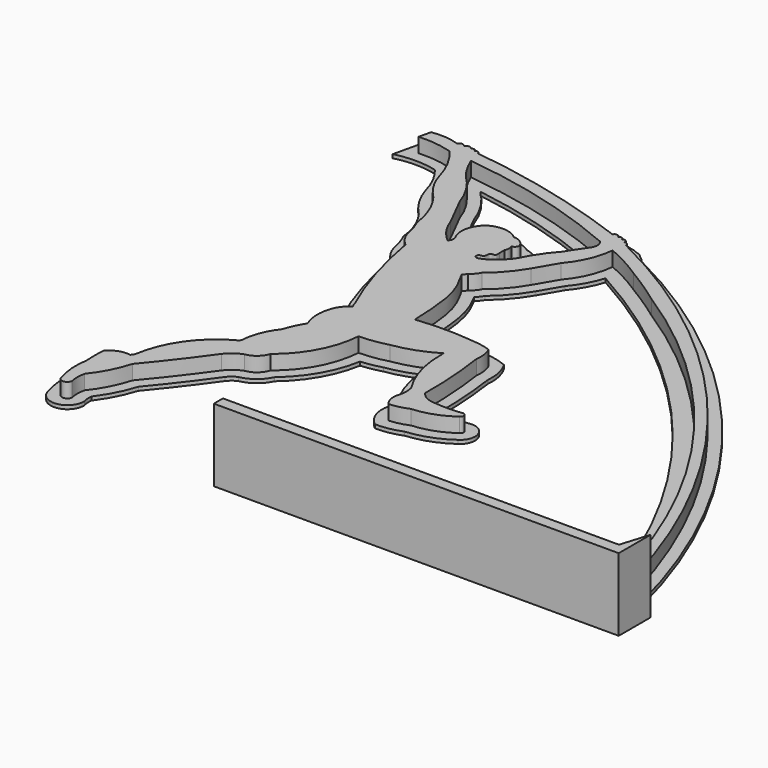
from build123d import *

# Parameters (mm, degrees)
F1_DEPTH = 2.5
F2_DEPTH = 0.5
F3_DEPTH = 10


# Not quite as in the source:
# - ends of sketch curves that miss each other by under 0.0002 mm in the source are joined
# - the dataset's text gives a spline's control points without its knots; the knots are read off the source's solid


with BuildPart() as f1:
    # F0 (on Top) → F1 (new body)
    with BuildSketch(Plane.XY):
        with BuildLine():
            ThreePointArc((-39.8229367736, 44.1013294606), (-37.4652443011, 44.0384179647), (-35.1560073833, 43.5587342062))
            ThreePointArc((-35.1560073833, 43.5587342062), (-33.4579822766, 41.1148254491), (-32.3751845495, 38.3429076368))
            ThreePointArc((-32.3751845495, 38.3429076368), (-31.3502645154, 36.0621986154), (-29.7918598256, 34.1068292029))
            ThreePointArc((-29.7918598256, 34.1068292029), (-28.2885518159, 31.4484118208), (-27.5291783241, 28.4902925114))
            ThreePointArc((-27.5291783241, 28.4902925114), (-26.9990197914, 27.1071797984), (-26.6612432485, 25.6649676596))
            ThreePointArc((-26.6612432485, 25.6649676596), (-26.0965046118, 24.5488660128), (-25.2444654097, 23.633092126))
            ThreePointArc((-25.2444654097, 23.633092126), (-23.5305341122, 16.3912786142), (-20.9041361566, 9.4282722799))
            ThreePointArc((-20.9041361566, 9.4282722799), (-20.8326707518, 9.1409651891), (-20.6576495277, 8.902176078))
            ThreePointArc((-20.6576495277, 8.902176078), (-21.6263146631, 8.0093254226), (-22.2124983376, 6.8295444526))
            ThreePointArc((-22.2124983376, 6.8295444526), (-22.4900033885, 4.788054511), (-22.0261043394, 2.7806960709))
            ThreePointArc((-22.0261043394, 2.7806960709), (-22.7702995051, 1.4335862053), (-23.3300869888, 0))
            ThreePointArc((-23.3300869888, 0), (-24.5116215298, -2.0072475649), (-25.10167519, -4.260446033))
            ThreePointArc((-25.10167519, -4.260446033), (-25.2008110189, -4.7928851197), (-25.6555593813, -5.0870334166))
            ThreePointArc((-25.6555593813, -5.0870334166), (-29.86125263, -8.9331377893), (-31.9792483024, -14.224117744))
            ThreePointArc((-31.9792483024, -14.224117744), (-32.102615125, -14.550216947), (-32.3352179546, -14.8099398509))
            ThreePointArc((-32.3352179546, -14.8099398509), (-33.8878424348, -14.9609911395), (-35.160557316, -15.863020019))
            ThreePointArc((-35.160557316, -15.863020019), (-35.2158724551, -17.3013725697), (-35.160557316, -18.7397251204))
            ThreePointArc((-35.160557316, -18.7397251204), (-35.2838018197, -21.1361854357), (-34.8258610521, -23.491711174))
            ThreePointArc((-34.8258610521, -23.491711174), (-34.1069338271, -24.1122417299), (-33.3880066022, -23.491711174))
            ThreePointArc((-33.3880066022, -23.491711174), (-33.5168735775, -22.400103951), (-33.3880066022, -21.308496728))
            ThreePointArc((-33.3880066022, -21.3084967281), (-31.8522050361, -18.9391366182), (-30.8167560275, -16.3122755386))
            ThreePointArc((-30.8167560275, -16.3122755386), (-27.7407229072, -12.4791780606), (-24.8122245337, -8.5322155185))
            ThreePointArc((-24.8122245337, -8.5322155185), (-23.9229409543, -7.6510921824), (-22.8184712103, -7.0617279464))
            ThreePointArc((-22.8184712104, -7.0617279464), (-21.491276404, -6.4601921468), (-20.6825484102, -5.2480657491))
            ThreePointArc((-20.6825484102, -5.2480657491), (-17.3317993937, -1.2028862045), (-15.8829957796, 3.8460705796))
            ThreePointArc((-15.8829957796, 3.8460705796), (-13.9186382863, 4.0008030408), (-11.9903566503, 4.4062317383))
            ThreePointArc((-11.9903566503, 4.4062317383), (-9.0377597077, 5.1571018461), (-6.2932519994, 6.4797174607))
            ThreePointArc((-6.2932519994, 6.4797174607), (-6.2856944043, 6.308996938), (-6.2700555864, 6.1388263134))
            ThreePointArc((-6.2700555864, 6.1388263134), (-5.7290502202, 1.9120041811), (-3.9806341619, -1.9740932741))
            ThreePointArc((-3.9806341619, -1.9740932742), (-3.8489454821, -2.9682730531), (-3.9806341619, -3.962452832))
            ThreePointArc((-3.9806341619, -3.962452832), (-4.0941358715, -5.2629547704), (-3.5290572438, -6.4397614982))
            ThreePointArc((-3.5290572438, -6.4397614982), (-2.208485014, -6.2406217831), (-0.9434746906, -5.8124669955))
            ThreePointArc((-0.9434746906, -5.8124669955), (1.7776886018, -5.2566320299), (4.2350820128, -3.962452832))
            ThreePointArc((4.2350820128, -3.962452832), (4.4423694361, -3.3533101685), (3.8401996851, -3.1265626187))
            ThreePointArc((3.8401996851, -3.1265626187), (1.9200998425, -3.2436876044), (0, -3.1265626187))
            ThreePointArc((0, -3.1265626187), (-1.1684109057, -2.7994599946), (-2.0577645744, -1.9740932742))
            ThreePointArc((-2.0577645744, -1.9740932742), (-2.1835629426, 2.8510857747), (-2.7043567721, 7.6497264021))
            ThreePointArc((-2.7043567721, 7.6497264021), (-2.6979040253, 8.9355969591), (-3.0520876401, 10.1717436714))
            ThreePointArc((-3.0520876402, 10.1717436714), (-4.332793982, 10.5090493439), (-5.6467727392, 10.6747106741))
            ThreePointArc((-5.6467727392, 10.6747106741), (-9.619203026, 10.9035585049), (-13.5916333127, 10.6747106741))
            add(Edge.make_bspline(
                [(-16.2312896614, 22.0125203762), (-15.5195201125, 20.7699562944), (-13.9004260765, 17.9422309955), (-13.7017233029, 13.2853516989), (-13.5916333127, 10.6747106741)],
                knots=[0, 0, 0, 0, 0.4394327051, 1, 1, 1, 1], degree=3))
            ThreePointArc((-16.2312896614, 22.0125203762), (-15.959177173, 22.2287700894), (-15.7865089656, 22.530423591))
            ThreePointArc((-15.7865089656, 22.530423591), (-15.1938705334, 23.0220818228), (-14.7743391242, 23.6677919163))
            ThreePointArc((-14.7743391242, 23.6677919163), (-12.8463325527, 25.5307631794), (-11.289681226, 27.7135842703))
            ThreePointArc((-11.289681226, 27.7135842703), (-10.4100338971, 29.2215741412), (-9.529445033, 30.7290143976))
            ThreePointArc((-9.529445033, 30.7290143976), (-7.8531159089, 33.4200131723), (-7.0535498671, 36.4879518747))
            ThreePointArc((-7.0535498671, 36.4879518747), (-4.4784790441, 35.2424402007), (-2.0295466339, 33.7642591823))
            ThreePointArc((-2.0295466339, 33.7642591823), (0.6201591638, 32.0998078893), (3.1916954177, 30.3169617893))
            ThreePointArc((3.1916954177, 30.3169617893), (28.684644436, 5.3376909151), (42.0442866041, -27.7587497425))
            Line((42.0442866041, -27.7587497425), (43.6340048841, -27.7587497425))
            Line((43.6340048841, -27.7587497425), (43.2501401956, -25.9507545681))
            ThreePointArc((43.2501401956, -25.9507545681), (25.6520284003, 11.9204246855), (-6.7084861254, 38.3158192924))
            ThreePointArc((-6.7084861254, 38.3158192924), (-6.8652378981, 38.6911658658), (-7.2716823309, 38.707262184))
            ThreePointArc((-7.2716823309, 38.707262184), (-7.4281605262, 39.1604792811), (-7.8963284894, 39.0569905337))
            ThreePointArc((-7.8963284894, 39.0569905337), (-8.1644501821, 39.4340035376), (-8.5762949973, 39.2232622378))
            ThreePointArc((-8.5762949973, 39.2232622378), (-8.9187752177, 39.6237059216), (-9.3860061412, 39.3801015097))
            ThreePointArc((-9.3860061412, 39.3801015097), (-20.745615536, 42.8862315911), (-32.4329830659, 45.0631822045))
            ThreePointArc((-32.4329830659, 45.0631822045), (-32.7032589825, 45.3661425954), (-33.0971016212, 45.2675421617))
            ThreePointArc((-33.0971016212, 45.2675421617), (-33.3311918709, 45.5738216629), (-33.6922671426, 45.4388030491))
            ThreePointArc((-33.6922671427, 45.4388030491), (-34.1690659606, 45.725806462), (-34.6458647786, 45.4388030491))
            ThreePointArc((-34.6458647786, 45.4388030491), (-35.1184636308, 45.734471068), (-35.5910624831, 45.4388030491))
            ThreePointArc((-35.5910624831, 45.4388030491), (-37.4934387451, 45.8368411623), (-39.4359203801, 45.7717652083))
            Line((-39.4359203801, 45.7717652083), (-39.8229367736, 44.1013294606))
        make_face()
        with BuildLine():
            ThreePointArc((-31.9367084144, 43.2399468127), (-20.4364233714, 41.0776813), (-9.3795687464, 37.2465047161))
            ThreePointArc((-9.3795687464, 37.2465047161), (-9.0591503252, 36.4552997594), (-9.2558916751, 35.6246577852))
            ThreePointArc((-9.2558916751, 35.6246577852), (-10.1914112813, 34.2828896711), (-11.0701493, 32.9032672229))
            ThreePointArc((-11.0701493, 32.9032672229), (-12.6550189015, 30.8835234947), (-13.9332200589, 28.6570064427))
            add(Edge.make_bspline(
                [(-16.1613304696, 28.3896197074), (-16.1629286922, 28.1762301343), (-16.0567322882, 27.5666666916), (-17.0562737858, 27.9215320494), (-16.7937765058, 26.5858814228), (-17.7948164446, 26.8632592396), (-17.6542923885, 25.1655984111), (-14.6178340155, 27.4848895748), (-13.9332200589, 28.6570064427)],
                knots=[0, 0, 0, 0, 0.1285053107, 0.2525069362, 0.402776315, 0.5314706313, 0.6581962639, 1, 1, 1, 1], degree=3))
            Line((-16.1613304696, 28.3896197074), (-16.1613304696, 29.2653576609))
            ThreePointArc((-16.1613304696, 29.2653576609), (-16.0071685922, 29.8589132326), (-16.1613304696, 30.4524688044))
            ThreePointArc((-16.1613304696, 30.4524688044), (-15.6822891013, 30.6627471064), (-15.5687948146, 31.173449215))
            ThreePointArc((-15.5687948146, 31.173449215), (-16.2444735736, 31.963289509), (-17.2396938456, 32.2631662931))
            ThreePointArc((-17.2396938456, 32.2631662931), (-19.276940378, 33.0633568611), (-21.3764754392, 32.4447851951))
            ThreePointArc((-21.3764754392, 32.4447851951), (-22.4637449003, 30.5775096234), (-22.2160693581, 28.4309938961))
            ThreePointArc((-22.2160693581, 28.4309938961), (-22.0368034912, 27.8016101926), (-22.342023403, 27.2227311874))
            ThreePointArc((-22.342023403, 27.2227311874), (-23.8214340034, 28.8526984955), (-24.8117185396, 30.8186043142))
            ThreePointArc((-24.8117185396, 30.8186043142), (-25.9053266059, 32.9870343231), (-26.9994337669, 35.1552125507))
            Line((-26.9994337669, 35.1552125507), (-26.9994337669, 35.1579960095))
            ThreePointArc((-26.9994337669, 35.1579960095), (-27.8821469058, 37.1802675534), (-29.1184878041, 39.007896035))
            ThreePointArc((-29.1184878041, 39.007896035), (-30.7630341358, 40.967139122), (-31.9367084144, 43.2399468127))
        make_face(mode=Mode.SUBTRACT)
    extrude(amount=F1_DEPTH)

    # F0 (on Top) → F2 (join)
    with BuildSketch(Plane.XY):
        with BuildLine():
            ThreePointArc((-39.8229367736, 44.1013294606), (-37.4652443011, 44.0384179647), (-35.1560073833, 43.5587342062))
            ThreePointArc((-35.1560073833, 43.5587342062), (-33.4579822766, 41.1148254491), (-32.3751845495, 38.3429076368))
            ThreePointArc((-32.3751845495, 38.3429076368), (-31.3502645154, 36.0621986154), (-29.7918598256, 34.1068292029))
            ThreePointArc((-29.7918598256, 34.1068292029), (-28.2885518159, 31.4484118208), (-27.5291783241, 28.4902925114))
            ThreePointArc((-27.5291783241, 28.4902925114), (-26.9990197914, 27.1071797984), (-26.6612432485, 25.6649676596))
            ThreePointArc((-26.6612432485, 25.6649676596), (-26.0965046118, 24.5488660128), (-25.2444654097, 23.633092126))
            ThreePointArc((-25.2444654097, 23.633092126), (-23.5305341122, 16.3912786142), (-20.9041361566, 9.4282722799))
            ThreePointArc((-20.9041361566, 9.4282722799), (-20.8326707518, 9.1409651891), (-20.6576495277, 8.902176078))
            ThreePointArc((-20.6576495277, 8.902176078), (-21.6263146631, 8.0093254226), (-22.2124983376, 6.8295444526))
            ThreePointArc((-22.2124983376, 6.8295444526), (-22.4900033885, 4.788054511), (-22.0261043394, 2.7806960709))
            ThreePointArc((-22.0261043394, 2.7806960709), (-22.7702995051, 1.4335862053), (-23.3300869888, 0))
            ThreePointArc((-23.3300869888, 0), (-24.5116215298, -2.0072475649), (-25.10167519, -4.260446033))
            ThreePointArc((-25.10167519, -4.260446033), (-25.2008110189, -4.7928851197), (-25.6555593813, -5.0870334166))
            ThreePointArc((-25.6555593813, -5.0870334166), (-29.86125263, -8.9331377893), (-31.9792483024, -14.224117744))
            ThreePointArc((-31.9792483024, -14.224117744), (-32.102615125, -14.550216947), (-32.3352179546, -14.8099398509))
            ThreePointArc((-32.3352179546, -14.8099398509), (-33.8878424348, -14.9609911395), (-35.160557316, -15.863020019))
            ThreePointArc((-35.160557316, -15.863020019), (-35.2158724551, -17.3013725697), (-35.160557316, -18.7397251204))
            ThreePointArc((-35.160557316, -18.7397251204), (-35.2838018197, -21.1361854357), (-34.8258610521, -23.491711174))
            ThreePointArc((-34.8258610521, -23.491711174), (-34.1069338271, -24.1122417299), (-33.3880066022, -23.491711174))
            ThreePointArc((-33.3880066022, -23.491711174), (-33.5168735775, -22.400103951), (-33.3880066022, -21.308496728))
            ThreePointArc((-33.3880066022, -21.3084967281), (-31.8522050361, -18.9391366182), (-30.8167560275, -16.3122755386))
            ThreePointArc((-30.8167560275, -16.3122755386), (-27.7407229072, -12.4791780606), (-24.8122245337, -8.5322155185))
            ThreePointArc((-24.8122245337, -8.5322155185), (-23.9229409543, -7.6510921824), (-22.8184712103, -7.0617279464))
            ThreePointArc((-22.8184712104, -7.0617279464), (-21.491276404, -6.4601921468), (-20.6825484102, -5.2480657491))
            ThreePointArc((-20.6825484102, -5.2480657491), (-17.3317993937, -1.2028862045), (-15.8829957796, 3.8460705796))
            ThreePointArc((-15.8829957796, 3.8460705796), (-13.9186382863, 4.0008030408), (-11.9903566503, 4.4062317383))
            ThreePointArc((-11.9903566503, 4.4062317383), (-9.0377597077, 5.1571018461), (-6.2932519994, 6.4797174607))
            ThreePointArc((-6.2932519994, 6.4797174607), (-6.2856944043, 6.308996938), (-6.2700555864, 6.1388263134))
            ThreePointArc((-6.2700555864, 6.1388263134), (-5.7290502202, 1.9120041811), (-3.9806341619, -1.9740932741))
            ThreePointArc((-3.9806341619, -1.9740932742), (-3.8489454821, -2.9682730531), (-3.9806341619, -3.962452832))
            ThreePointArc((-3.9806341619, -3.962452832), (-4.0941358715, -5.2629547704), (-3.5290572438, -6.4397614982))
            ThreePointArc((-3.5290572438, -6.4397614982), (-2.208485014, -6.2406217831), (-0.9434746906, -5.8124669955))
            ThreePointArc((-0.9434746906, -5.8124669955), (1.7776886018, -5.2566320299), (4.2350820128, -3.962452832))
            ThreePointArc((4.2350820128, -3.962452832), (4.4423694361, -3.3533101685), (3.8401996851, -3.1265626187))
            ThreePointArc((3.8401996851, -3.1265626187), (1.9200998425, -3.2436876044), (0, -3.1265626187))
            ThreePointArc((0, -3.1265626187), (-1.1684109057, -2.7994599946), (-2.0577645744, -1.9740932742))
            ThreePointArc((-2.0577645744, -1.9740932742), (-2.1835629426, 2.8510857747), (-2.7043567721, 7.6497264021))
            ThreePointArc((-2.7043567721, 7.6497264021), (-2.6979040253, 8.9355969591), (-3.0520876401, 10.1717436714))
            ThreePointArc((-3.0520876402, 10.1717436714), (-4.332793982, 10.5090493439), (-5.6467727392, 10.6747106741))
            ThreePointArc((-5.6467727392, 10.6747106741), (-9.619203026, 10.9035585049), (-13.5916333127, 10.6747106741))
            add(Edge.make_bspline(
                [(-16.2312896614, 22.0125203762), (-15.5195201125, 20.7699562944), (-13.9004260765, 17.9422309955), (-13.7017233029, 13.2853516989), (-13.5916333127, 10.6747106741)],
                knots=[0, 0, 0, 0, 0.4394327051, 1, 1, 1, 1], degree=3))
            ThreePointArc((-16.2312896614, 22.0125203762), (-15.959177173, 22.2287700894), (-15.7865089656, 22.530423591))
            ThreePointArc((-15.7865089656, 22.530423591), (-15.1938705334, 23.0220818228), (-14.7743391242, 23.6677919163))
            ThreePointArc((-14.7743391242, 23.6677919163), (-12.8463325527, 25.5307631794), (-11.289681226, 27.7135842703))
            ThreePointArc((-11.289681226, 27.7135842703), (-10.4100338971, 29.2215741412), (-9.529445033, 30.7290143976))
            ThreePointArc((-9.529445033, 30.7290143976), (-7.8531159089, 33.4200131723), (-7.0535498671, 36.4879518747))
            ThreePointArc((-7.0535498671, 36.4879518747), (-4.4784790441, 35.2424402007), (-2.0295466339, 33.7642591823))
            ThreePointArc((-2.0295466339, 33.7642591823), (0.6201591638, 32.0998078893), (3.1916954177, 30.3169617893))
            ThreePointArc((3.1916954177, 30.3169617893), (28.684644436, 5.3376909151), (42.0442866041, -27.7587497425))
            Line((42.0442866041, -27.7587497425), (43.6340048841, -27.7587497425))
            Line((43.6340048841, -27.7587497425), (43.2501401956, -25.9507545681))
            ThreePointArc((43.2501401956, -25.9507545681), (25.6520284003, 11.9204246855), (-6.7084861254, 38.3158192924))
            ThreePointArc((-6.7084861254, 38.3158192924), (-6.8652378981, 38.6911658658), (-7.2716823309, 38.707262184))
            ThreePointArc((-7.2716823309, 38.707262184), (-7.4281605262, 39.1604792811), (-7.8963284894, 39.0569905337))
            ThreePointArc((-7.8963284894, 39.0569905337), (-8.1644501821, 39.4340035376), (-8.5762949973, 39.2232622378))
            ThreePointArc((-8.5762949973, 39.2232622378), (-8.9187752177, 39.6237059216), (-9.3860061412, 39.3801015097))
            ThreePointArc((-9.3860061412, 39.3801015097), (-20.745615536, 42.8862315911), (-32.4329830659, 45.0631822045))
            ThreePointArc((-32.4329830659, 45.0631822045), (-32.7032589825, 45.3661425954), (-33.0971016212, 45.2675421617))
            ThreePointArc((-33.0971016212, 45.2675421617), (-33.3311918709, 45.5738216629), (-33.6922671426, 45.4388030491))
            ThreePointArc((-33.6922671427, 45.4388030491), (-34.1690659606, 45.725806462), (-34.6458647786, 45.4388030491))
            ThreePointArc((-34.6458647786, 45.4388030491), (-35.1184636308, 45.734471068), (-35.5910624831, 45.4388030491))
            ThreePointArc((-35.5910624831, 45.4388030491), (-37.4934387451, 45.8368411623), (-39.4359203801, 45.7717652083))
            Line((-39.4359203801, 45.7717652083), (-39.8229367736, 44.1013294606))
        make_face()
        with BuildLine():
            ThreePointArc((-31.9367084144, 43.2399468127), (-20.4364233714, 41.0776813), (-9.3795687464, 37.2465047161))
            ThreePointArc((-9.3795687464, 37.2465047161), (-9.0591503252, 36.4552997594), (-9.2558916751, 35.6246577852))
            ThreePointArc((-9.2558916751, 35.6246577852), (-10.1914112813, 34.2828896711), (-11.0701493, 32.9032672229))
            ThreePointArc((-11.0701493, 32.9032672229), (-12.6550189015, 30.8835234947), (-13.9332200589, 28.6570064427))
            add(Edge.make_bspline(
                [(-16.1613304696, 28.3896197074), (-16.1629286922, 28.1762301343), (-16.0567322882, 27.5666666916), (-17.0562737858, 27.9215320494), (-16.7937765058, 26.5858814228), (-17.7948164446, 26.8632592396), (-17.6542923885, 25.1655984111), (-14.6178340155, 27.4848895748), (-13.9332200589, 28.6570064427)],
                knots=[0, 0, 0, 0, 0.1285053107, 0.2525069362, 0.402776315, 0.5314706313, 0.6581962639, 1, 1, 1, 1], degree=3))
            Line((-16.1613304696, 28.3896197074), (-16.1613304696, 29.2653576609))
            ThreePointArc((-16.1613304696, 29.2653576609), (-16.0071685922, 29.8589132326), (-16.1613304696, 30.4524688044))
            ThreePointArc((-16.1613304696, 30.4524688044), (-15.6822891013, 30.6627471064), (-15.5687948146, 31.173449215))
            ThreePointArc((-15.5687948146, 31.173449215), (-16.2444735736, 31.963289509), (-17.2396938456, 32.2631662931))
            ThreePointArc((-17.2396938456, 32.2631662931), (-19.276940378, 33.0633568611), (-21.3764754392, 32.4447851951))
            ThreePointArc((-21.3764754392, 32.4447851951), (-22.4637449003, 30.5775096234), (-22.2160693581, 28.4309938961))
            ThreePointArc((-22.2160693581, 28.4309938961), (-22.0368034912, 27.8016101926), (-22.342023403, 27.2227311874))
            ThreePointArc((-22.342023403, 27.2227311874), (-23.8214340034, 28.8526984955), (-24.8117185396, 30.8186043142))
            ThreePointArc((-24.8117185396, 30.8186043142), (-25.9053266059, 32.9870343231), (-26.9994337669, 35.1552125507))
            Line((-26.9994337669, 35.1552125507), (-26.9994337669, 35.1579960095))
            ThreePointArc((-26.9994337669, 35.1579960095), (-27.8821469058, 37.1802675534), (-29.1184878041, 39.007896035))
            ThreePointArc((-29.1184878041, 39.007896035), (-30.7630341358, 40.967139122), (-31.9367084144, 43.2399468127))
        make_face(mode=Mode.SUBTRACT)
        with BuildLine():
            ThreePointArc((-32.3751845495, 38.3429076368), (-33.4579822766, 41.1148254491), (-35.1560073833, 43.5587342062))
            ThreePointArc((-35.1560073833, 43.5587342062), (-37.4652443011, 44.0384179647), (-39.8229367736, 44.1013294606))
            Line((-39.8229367736, 44.1013294606), (-39.4359203801, 45.7717652083))
            ThreePointArc((-39.4359203801, 45.7717652083), (-37.4934387451, 45.8368411623), (-35.5910624831, 45.4388030491))
            ThreePointArc((-35.5910624831, 45.4388030491), (-35.1184636308, 45.734471068), (-34.6458647786, 45.4388030491))
            ThreePointArc((-34.6458647786, 45.4388030491), (-34.1690659606, 45.725806462), (-33.6922671427, 45.4388030491))
            ThreePointArc((-33.6922671427, 45.4388030491), (-33.3311918709, 45.5738216629), (-33.0971016212, 45.2675421617))
            ThreePointArc((-33.0971016212, 45.2675421617), (-32.7032589825, 45.3661425954), (-32.4329830659, 45.0631822045))
            ThreePointArc((-32.4329830659, 45.0631822045), (-20.745615536, 42.8862315911), (-9.3860061412, 39.3801015097))
            ThreePointArc((-9.3860061412, 39.3801015097), (-8.9187752177, 39.6237059216), (-8.5762949973, 39.2232622378))
            ThreePointArc((-8.5762949973, 39.2232622378), (-8.1644501821, 39.4340035376), (-7.8963284894, 39.0569905337))
            ThreePointArc((-7.8963284894, 39.0569905337), (-7.4281605262, 39.1604792811), (-7.2716823309, 38.707262184))
            ThreePointArc((-7.2716823309, 38.707262184), (-6.8652378981, 38.6911658658), (-6.7084861254, 38.3158192924))
            ThreePointArc((-6.7084861254, 38.3158192924), (25.6520284003, 11.9204246855), (43.2501401956, -25.9507545681))
            Line((43.2501401956, -25.9507545681), (43.6340048841, -27.7587497425))
            Line((43.6340048841, -27.7587497425), (45.2058374977, -27.7587497425))
            ThreePointArc((45.2058374977, -27.7587497425), (27.7383372604, 11.7655763293), (-5.452482748, 39.4360548786))
            ThreePointArc((-5.452482748, 39.4360548786), (-5.7471592831, 39.7902042097), (-6.1170118114, 40.0649133585))
            ThreePointArc((-6.1170118114, 40.0649133585), (-6.6347697136, 40.5066449859), (-7.2739788579, 40.7403365469))
            ThreePointArc((-7.2739788579, 40.7403365469), (-7.6970818912, 40.9255829398), (-8.1522197382, 41.004208274))
            ThreePointArc((-8.1522197382, 41.004208274), (-8.848843866, 41.1882238858), (-9.56527135, 41.1115519798))
            ThreePointArc((-9.56527135, 41.1115519798), (-20.4435268265, 44.4210164676), (-31.6162907237, 46.5324956426))
            ThreePointArc((-31.6162907237, 46.5324956426), (-32.0468133147, 46.7871695777), (-32.5278726763, 46.9242476765))
            ThreePointArc((-32.5278726763, 46.9242476765), (-32.9582820792, 47.0913819274), (-33.4164017239, 47.1489362767))
            ThreePointArc((-33.4164017239, 47.1489362767), (-34.0146082635, 47.2826240527), (-34.6259485874, 47.2380539517))
            ThreePointArc((-34.6259485874, 47.2380539517), (-35.2628906299, 47.2919701599), (-35.886297231, 47.1506678853))
            ThreePointArc((-35.886297231, 47.1506678853), (-38.3140447945, 47.4289050593), (-40.7341906472, 47.0908692496))
            Line((-40.7341906472, 47.0908692496), (-41.8656741024, 42.207173253))
            ThreePointArc((-41.8656741024, 42.207173253), (-38.9503145165, 42.564533406), (-36.0378569834, 42.1842454735))
            ThreePointArc((-36.0378569834, 42.1842454735), (-34.7272004395, 40.1688384337), (-33.8794820827, 37.9191585231))
            ThreePointArc((-33.8794820827, 37.9191585231), (-32.7263503484, 35.3182167514), (-30.973262246, 33.0773925723))
            ThreePointArc((-30.973262246, 33.0773925723), (-29.6722520676, 30.6973942824), (-29.0538824219, 28.0564402265))
            ThreePointArc((-29.0538824219, 28.0564402265), (-28.5122969659, 26.7115604502), (-28.1853835888, 25.2990647643))
            ThreePointArc((-28.1853835888, 25.2990647643), (-27.5876681367, 23.9769704143), (-26.6914309452, 22.8359374923))
            ThreePointArc((-26.6914309452, 22.8359374923), (-25.0312798268, 15.9557985517), (-22.5673474771, 9.3209322415))
            ThreePointArc((-22.5673474771, 9.3209322415), (-23.2523309951, 8.3693472354), (-23.7063383608, 7.2883320848))
            ThreePointArc((-23.7063383608, 7.2883320848), (-24.0582187667, 5.12095476), (-23.7480069459, 2.9472222754))
            ThreePointArc((-23.7480069459, 2.9472222754), (-24.2904247504, 1.8663780777), (-24.7315812644, 0.7404019747))
            ThreePointArc((-24.7315812644, 0.7404019747), (-25.9645033138, -1.4318054839), (-26.6225640587, -3.8412739065))
            ThreePointArc((-26.6225640587, -3.8412739065), (-30.9943894305, -7.8290241894), (-33.3863369365, -13.2413801024))
            ThreePointArc((-33.3863369365, -13.2413801024), (-35.2594198192, -13.9029816809), (-36.6787194883, -15.2928538272))
            ThreePointArc((-36.6787194883, -15.2928538272), (-36.7758112269, -16.978987371), (-36.7323411306, -18.6673544767))
            ThreePointArc((-36.7323411306, -18.6673544767), (-36.8387885006, -21.2962368232), (-36.3421249699, -23.8799703179))
            ThreePointArc((-36.3421249699, -23.8799703179), (-33.820799216, -25.6567891072), (-31.8189464067, -23.3101417333))
            ThreePointArc((-31.8189464067, -23.3101417333), (-31.9445706599, -22.6474470608), (-31.9250842678, -21.9732319894))
            ThreePointArc((-31.9250842678, -21.9732319894), (-30.4502898772, -19.6295898297), (-29.4093048474, -17.0636538922))
            ThreePointArc((-29.4093048474, -17.0636538922), (-26.411434212, -13.3140445309), (-23.5527787293, -9.4572469552))
            ThreePointArc((-23.5527787293, -9.4572469552), (-23.0365442818, -8.93943949), (-22.4024724628, -8.5753302974))
            ThreePointArc((-22.4024724628, -8.5753302974), (-20.6035319363, -7.7522229199), (-19.3785829682, -6.1987774596))
            ThreePointArc((-19.3785829682, -6.1987774596), (-16.1800605751, -2.3512004909), (-14.4920808787, 2.3589076367))
            ThreePointArc((-14.4920808787, 2.3589076367), (-13.0668512986, 2.556937913), (-11.6636462069, 2.8755455354))
            ThreePointArc((-11.6636462069, 2.8755455354), (-9.6619704163, 3.3140624973), (-7.7284862998, 3.9927688166))
            ThreePointArc((-7.7284862998, 3.9927688166), (-6.947589186, 0.5806614985), (-5.4449786352, -2.5807366392))
            ThreePointArc((-5.4449786352, -2.5807366392), (-5.4127136383, -3.0439076402), (-5.4759436587, -3.5038754334))
            ThreePointArc((-5.4759436587, -3.5038754334), (-5.5269748981, -5.9775428101), (-4.1240598173, -8.0155476566))
            ThreePointArc((-4.1240598173, -8.0155476566), (-2.3159220901, -7.8611695582), (-0.5740240618, -7.3522629885))
            ThreePointArc((-0.5740240618, -7.3522629885), (2.3952568572, -6.6947770134), (5.0850753832, -5.2756951691))
            ThreePointArc((5.0850753832, -5.2756951691), (5.8862838329, -2.7551186393), (3.5109020504, -1.5920182954))
            ThreePointArc((3.5109020504, -1.5920182954), (1.8092215943, -1.6807557673), (0.1091299886, -1.5655201562))
            ThreePointArc((0.1091299886, -1.5655201562), (-0.2045086726, -1.521651177), (-0.4893761207, -1.3832884863))
            ThreePointArc((-0.4893761207, -1.3832884863), (-0.6382145312, 3.1539307847), (-1.127334416, 7.667163919))
            ThreePointArc((-1.127334416, 7.667163919), (-1.2328321987, 9.6150688442), (-1.9474209279, 11.4302344917))
            ThreePointArc((-1.9474209279, 11.4302344917), (-3.6967223474, 11.972074632), (-5.5095180192, 12.2317244838))
            ThreePointArc((-5.5095180192, 12.2317244838), (-8.8034333765, 12.4568540319), (-12.1041516249, 12.3805602624))
            add(Edge.make_bspline(
                [(-14.2767808193, 21.7257843197), (-14.2701097331, 21.7135252149), (-14.0558784074, 21.3191779721), (-13.6365212944, 20.5036921305), (-13.1736655888, 19.3743343129), (-12.8636668441, 18.374726434), (-12.607843269, 17.3238548871), (-12.3817884692, 15.9584819349), (-12.2108686107, 14.2479726229), (-12.1377619618, 13.0422985102), (-12.1060701141, 12.4187126371), (-12.1041516249, 12.3805602624)],
                knots=[0.1209830334, 0.1209830334, 0.1209830334, 0.1209830334, 0.125, 0.25, 0.375, 0.4375, 0.5, 0.625, 0.75, 0.875, 0.8831451051, 0.8831451051, 0.8831451051, 0.8831451051], degree=3))
            ThreePointArc((-14.2767808193, 21.7257843197), (-13.8723124268, 22.1672806089), (-13.5360840782, 22.6627264998))
            ThreePointArc((-13.5360840782, 22.6627264998), (-11.5514069806, 24.6413510536), (-9.9367378319, 26.9319278034))
            ThreePointArc((-9.9367378319, 26.9319278034), (-9.0932448247, 28.3779727818), (-8.2488855607, 29.8235121157))
            ThreePointArc((-8.2488855607, 29.8235121157), (-6.9220531656, 31.7683036736), (-5.9971213215, 33.9332977826))
            ThreePointArc((-5.9971213215, 33.9332977826), (23.9136010879, 8.0349743467), (40.7713526483, -27.7587497425))
            Line((40.7713526483, -27.7587497425), (42.0442866041, -27.7587497425))
            ThreePointArc((42.0442866041, -27.7587497425), (28.684644436, 5.3376909151), (3.1916954177, 30.3169617893))
            ThreePointArc((3.1916954177, 30.3169617893), (0.6201591638, 32.0998078893), (-2.0295466339, 33.7642591823))
            ThreePointArc((-2.0295466339, 33.7642591823), (-4.4784790441, 35.2424402007), (-7.0535498671, 36.4879518747))
            ThreePointArc((-7.0535498671, 36.4879518747), (-7.8531159089, 33.4200131723), (-9.529445033, 30.7290143976))
            ThreePointArc((-9.529445033, 30.7290143976), (-10.4100338971, 29.2215741412), (-11.289681226, 27.7135842703))
            ThreePointArc((-11.289681226, 27.7135842703), (-12.8463325527, 25.5307631794), (-14.7743391242, 23.6677919163))
            ThreePointArc((-14.7743391242, 23.6677919163), (-15.1938705334, 23.0220818228), (-15.7865089656, 22.530423591))
            ThreePointArc((-15.7865089656, 22.530423591), (-15.959177173, 22.2287700894), (-16.2312896614, 22.0125203762))
            add(Edge.make_bspline(
                [(-16.2312896614, 22.0125203762), (-15.5195201125, 20.7699562944), (-13.9004260765, 17.9422309955), (-13.7017233029, 13.2853516989), (-13.5916333127, 10.6747106741)],
                knots=[0, 0, 0, 0, 0.4394327051, 1, 1, 1, 1], degree=3))
            ThreePointArc((-13.5916333127, 10.6747106741), (-9.619203026, 10.9035585049), (-5.6467727392, 10.6747106741))
            ThreePointArc((-5.6467727392, 10.6747106741), (-4.332793982, 10.5090493439), (-3.0520876402, 10.1717436714))
            ThreePointArc((-3.0520876402, 10.1717436714), (-2.6979040253, 8.9355969591), (-2.7043567721, 7.6497264021))
            ThreePointArc((-2.7043567721, 7.6497264021), (-2.1835629426, 2.8510857747), (-2.0577645744, -1.9740932742))
            ThreePointArc((-2.0577645744, -1.9740932742), (-1.1684109057, -2.7994599946), (0, -3.1265626187))
            ThreePointArc((0, -3.1265626187), (1.9200998425, -3.2436876044), (3.8401996851, -3.1265626187))
            ThreePointArc((3.8401996851, -3.1265626187), (4.4423694361, -3.3533101685), (4.2350820128, -3.962452832))
            ThreePointArc((4.2350820128, -3.962452832), (1.7776886018, -5.2566320299), (-0.9434746906, -5.8124669955))
            ThreePointArc((-0.9434746906, -5.8124669955), (-2.208485014, -6.2406217831), (-3.5290572438, -6.4397614982))
            ThreePointArc((-3.5290572438, -6.4397614982), (-4.0941358715, -5.2629547704), (-3.9806341619, -3.962452832))
            ThreePointArc((-3.9806341619, -3.962452832), (-3.8489454821, -2.9682730531), (-3.9806341619, -1.9740932742))
            ThreePointArc((-3.9806341619, -1.9740932742), (-5.7290502202, 1.9120041811), (-6.2700555864, 6.1388263134))
            ThreePointArc((-6.2700555864, 6.1388263134), (-6.2856944043, 6.308996938), (-6.2932519994, 6.4797174607))
            ThreePointArc((-6.2932519994, 6.4797174607), (-9.0377597077, 5.1571018461), (-11.9903566503, 4.4062317383))
            ThreePointArc((-11.9903566503, 4.4062317383), (-13.9186382863, 4.0008030408), (-15.8829957796, 3.8460705796))
            ThreePointArc((-15.8829957796, 3.8460705796), (-17.3317993937, -1.2028862045), (-20.6825484102, -5.2480657491))
            ThreePointArc((-20.6825484102, -5.2480657491), (-21.491276404, -6.4601921468), (-22.8184712104, -7.0617279464))
            ThreePointArc((-22.8184712104, -7.0617279464), (-23.9229409543, -7.6510921824), (-24.8122245337, -8.5322155185))
            ThreePointArc((-24.8122245337, -8.5322155185), (-27.7407229072, -12.4791780606), (-30.8167560275, -16.3122755386))
            ThreePointArc((-30.8167560275, -16.3122755386), (-31.8522050361, -18.9391366182), (-33.3880066022, -21.3084967281))
            ThreePointArc((-33.3880066022, -21.3084967281), (-33.5168735775, -22.400103951), (-33.3880066022, -23.491711174))
            ThreePointArc((-33.3880066022, -23.491711174), (-34.1069338271, -24.1122417299), (-34.8258610521, -23.491711174))
            ThreePointArc((-34.8258610521, -23.491711174), (-35.2838018197, -21.1361854357), (-35.160557316, -18.7397251204))
            ThreePointArc((-35.160557316, -18.7397251204), (-35.2158724551, -17.3013725697), (-35.160557316, -15.863020019))
            ThreePointArc((-35.160557316, -15.863020019), (-33.8878424348, -14.9609911395), (-32.3352179546, -14.8099398509))
            ThreePointArc((-32.3352179546, -14.8099398509), (-32.102615125, -14.550216947), (-31.9792483024, -14.224117744))
            ThreePointArc((-31.9792483024, -14.224117744), (-29.86125263, -8.9331377893), (-25.6555593813, -5.0870334166))
            ThreePointArc((-25.6555593813, -5.0870334166), (-25.2008110189, -4.7928851197), (-25.10167519, -4.260446033))
            ThreePointArc((-25.10167519, -4.260446033), (-24.5116215298, -2.0072475649), (-23.3300869888, 0))
            ThreePointArc((-23.3300869888, 0), (-22.7702995051, 1.4335862053), (-22.0261043394, 2.7806960709))
            ThreePointArc((-22.0261043394, 2.7806960709), (-22.4900033885, 4.788054511), (-22.2124983376, 6.8295444526))
            ThreePointArc((-22.2124983376, 6.8295444526), (-21.6263146631, 8.0093254226), (-20.6576495277, 8.902176078))
            ThreePointArc((-20.6576495277, 8.902176078), (-20.8326707518, 9.1409651891), (-20.9041361566, 9.4282722799))
            ThreePointArc((-20.9041361566, 9.4282722799), (-23.5305341122, 16.3912786142), (-25.2444654097, 23.633092126))
            ThreePointArc((-25.2444654097, 23.633092126), (-26.0965046118, 24.5488660128), (-26.6612432485, 25.6649676596))
            ThreePointArc((-26.6612432485, 25.6649676596), (-26.9990197914, 27.1071797984), (-27.5291783241, 28.4902925114))
            ThreePointArc((-27.5291783241, 28.4902925114), (-28.2885518159, 31.4484118208), (-29.7918598256, 34.1068292029))
            ThreePointArc((-29.7918598256, 34.1068292029), (-31.3502645154, 36.0621986154), (-32.3751845495, 38.3429076368))
        make_face()
        with BuildLine():
            ThreePointArc((-9.2558916751, 35.6246577852), (-9.0591503252, 36.4552997594), (-9.3795687464, 37.2465047161))
            ThreePointArc((-9.3795687464, 37.2465047161), (-20.4364233714, 41.0776813), (-31.9367084144, 43.2399468127))
            ThreePointArc((-31.9367084144, 43.2399468127), (-30.7630341358, 40.967139122), (-29.1184878041, 39.007896035))
            ThreePointArc((-29.1184878041, 39.007896035), (-27.8821469058, 37.1802675534), (-26.9994337669, 35.1579960095))
            Line((-26.9994337669, 35.1579960095), (-26.9994337669, 35.1552125507))
            ThreePointArc((-26.9994337669, 35.1552125507), (-25.9053266059, 32.9870343231), (-24.8117185396, 30.8186043142))
            ThreePointArc((-24.8117185396, 30.8186043142), (-23.8214340034, 28.8526984955), (-22.342023403, 27.2227311874))
            ThreePointArc((-22.342023403, 27.2227311874), (-22.0368034912, 27.8016101926), (-22.2160693581, 28.4309938961))
            ThreePointArc((-22.2160693581, 28.4309938961), (-22.4637449003, 30.5775096234), (-21.3764754392, 32.4447851951))
            ThreePointArc((-21.3764754392, 32.4447851951), (-19.276940378, 33.0633568611), (-17.2396938456, 32.2631662931))
            ThreePointArc((-17.2396938456, 32.2631662931), (-16.2444735736, 31.963289509), (-15.5687948146, 31.173449215))
            ThreePointArc((-15.5687948146, 31.173449215), (-15.6822891013, 30.6627471064), (-16.1613304696, 30.4524688044))
            ThreePointArc((-16.1613304696, 30.4524688044), (-16.0071685922, 29.8589132326), (-16.1613304696, 29.2653576609))
            Line((-16.1613304696, 29.2653576609), (-16.1613304696, 28.3896197074))
            add(Edge.make_bspline(
                [(-16.1613304696, 28.3896197074), (-16.1629286922, 28.1762301343), (-16.0567322882, 27.5666666916), (-17.0562737858, 27.9215320494), (-16.7937765058, 26.5858814228), (-17.7948164446, 26.8632592396), (-17.6542923885, 25.1655984111), (-14.6178340155, 27.4848895748), (-13.9332200589, 28.6570064427)],
                knots=[0, 0, 0, 0, 0.1285053107, 0.2525069362, 0.402776315, 0.5314706313, 0.6581962639, 1, 1, 1, 1], degree=3))
            ThreePointArc((-13.9332200589, 28.6570064427), (-12.6550189015, 30.8835234947), (-11.0701493, 32.9032672229))
            ThreePointArc((-11.0701493, 32.9032672229), (-10.1914112813, 34.2828896711), (-9.2558916751, 35.6246577852))
        make_face()
        with BuildLine():
            ThreePointArc((-16.6433087488, 33.770686071), (-19.5112055285, 34.6283487564), (-22.3473612527, 33.6709366567))
            ThreePointArc((-22.3473612527, 33.6709366567), (-23.086312061, 32.8883738833), (-23.6400962981, 31.9654568719))
            ThreePointArc((-23.6400962981, 31.9654568719), (-24.5954669432, 33.8596336323), (-25.5512183728, 35.7536182875))
            ThreePointArc((-25.5512183728, 35.7536182875), (-26.5648455472, 38.0264931569), (-27.9750012669, 40.0770689459))
            ThreePointArc((-27.9750012669, 40.0770689459), (-28.5468940203, 40.6583071689), (-29.0695479045, 41.2841922308))
            ThreePointArc((-29.0695479045, 41.2841922308), (-19.778040958, 39.2780050517), (-10.8008651537, 36.1527525956))
            ThreePointArc((-10.8008651537, 36.1527525956), (-11.5841191942, 35.0100441638), (-12.3280956839, 33.8413832058))
            ThreePointArc((-12.3280956839, 33.8413832058), (-13.2366512022, 32.7470752836), (-14.0625146519, 31.5890888758))
            ThreePointArc((-14.0625146519, 31.5890888758), (-14.0801930931, 31.6507587457), (-14.0997113341, 31.7118712518))
            ThreePointArc((-14.0997113341, 31.7118712518), (-15.108363071, 33.0663880144), (-16.6433087488, 33.770686071))
        make_face(mode=Mode.SUBTRACT)
    extrude(amount=F2_DEPTH)

    # F0 (on Top) → F3 (join)
    with BuildSketch(Plane.XY):
        Polygon((45.2058374977, -27.7587497425), (43.6340048841, -27.7587497425), (42.0442866041, -27.7587497425), (40.7713526483, -27.7587497425), (-9.2286473517, -27.7587497425), (-9.2286473517, -29.3212497425), (46.4224337241, -29.3212497425), (46.4224337241, -27.7587497425), (46.4224337241, -23.8347464923), align=None)
    extrude(amount=F3_DEPTH)


solid = f1.part
